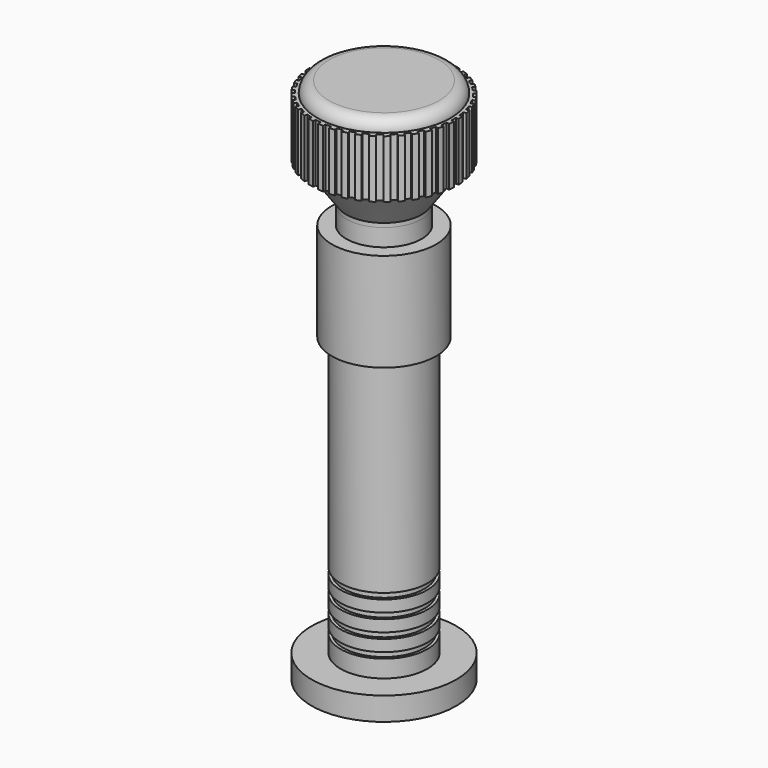
from build123d import *

# Parameters (mm, degrees)
F0_R             = 12.5
F1_DEPTH         = 4
F2_R             = 7.5
F3_DEPTH         = 3
F4_R             = 7
F5_DEPTH         = 1
F6_R             = 7.5
F7_DEPTH         = 2
F8_R             = 7
F9_DEPTH         = 1
F10_R            = 7.5
F11_DEPTH        = 2
F12_R            = 7
F13_DEPTH        = 1
F14_R            = 7.5
F15_DEPTH        = 2
F16_R            = 7
F17_DEPTH        = 1
F18_R            = 7.5
F19_DEPTH        = 35
F20_R            = 9
F21_DEPTH        = 17
F22_R            = 6.5
F23_DEPTH        = 3
F24_R            = 11
F25_DEPTH        = 7
F26_R            = 12.5
F27_DEPTH        = 10
F28_S6_R         = 6.5
F28_T7_DEPTH     = 17
F29_R            = 11.5
F30_DEPTH        = 2
F31_R            = 1.99999
F33_DEPTH        = 25
F33_COPIES_COUNT = 40
F34_R            = 2
F35_DEPTH        = 10


# Not quite as in the source:
# - a fillet or chamfer that OpenCascade refuses, or shapes differently, is made with other operations: its cross-section is extruded or revolved along the edge and cut away or added
# - a fillet or chamfer is up to 0.001 mm smaller than in the source, because OpenCascade refuses the exact size
# - a pattern or mirror of a feature is missing from the dataset's text; its kind, count and spacing are read off the source's solid


with BuildPart() as f1:
    # F0 (on Top) → F1 (new body)
    with BuildSketch(Plane.XY):
        Circle(F0_R)
    extrude(amount=F1_DEPTH)

    # F2 (on face) → F3 (join)
    with BuildSketch(Plane.XY.offset(4)):
        Circle(F2_R)
    extrude(amount=F3_DEPTH)

    # F4 (on face) → F5 (join)
    with BuildSketch(Plane.XY.offset(7)):
        Circle(F4_R)
    extrude(amount=F5_DEPTH)

    # F6 (on face) → F7 (join)
    with BuildSketch(Plane.XY.offset(8)):
        Circle(F6_R)
    extrude(amount=F7_DEPTH)

    # F8 (on face) → F9 (join)
    with BuildSketch(Plane.XY.offset(10)):
        Circle(F8_R)
    extrude(amount=F9_DEPTH)

    # F10 (on face) → F11 (join)
    with BuildSketch(Plane.XY.offset(11)):
        Circle(F10_R)
    extrude(amount=F11_DEPTH)

    # F12 (on face) → F13 (join)
    with BuildSketch(Plane.XY.offset(13)):
        Circle(F12_R)
    extrude(amount=F13_DEPTH)

    # F14 (on face) → F15 (join)
    with BuildSketch(Plane.XY.offset(14)):
        Circle(F14_R)
    extrude(amount=F15_DEPTH)

    # F16 (on face) → F17 (join)
    with BuildSketch(Plane.XY.offset(16)):
        Circle(F16_R)
    extrude(amount=F17_DEPTH)

    # F18 (on face) → F19 (join)
    with BuildSketch(Plane.XY.offset(17)):
        Circle(F18_R)
    extrude(amount=F19_DEPTH)

    # F20 (on face) → F21 (join)
    with BuildSketch(Plane.XY.offset(52)):
        Circle(F20_R)
    extrude(amount=F21_DEPTH)

    # F22 (on face) → F23 (join)
    with BuildSketch(Plane.XY.offset(69)):
        Circle(F22_R)
    extrude(amount=F23_DEPTH)

    # F24 (on face) → F25 (join)
    with BuildSketch(Plane.XY.offset(72)):
        Circle(F24_R)
    extrude(amount=F25_DEPTH)

    # F26 (on face) → F27 (join)
    with BuildSketch(Plane.XY.offset(79)):
        Circle(F26_R)
    extrude(amount=F27_DEPTH)

    # F28: chamfer of 7 x 5 on 1 edges, made by hand


with BuildPart() as f28_tool2:
    # F28_s3 → F28_t4 (revolve)
    with BuildSketch(Plane.XZ):
        Polygon((11, 79), (6, 72), (11, 72), align=None)
    revolve(axis=Axis((0, 0, 72), (0, 0, 1)))

    split(bisect_by=Plane.XY.offset(79), keep=Keep.BOTTOM)

    # F28_s6 → F28_t7 (cut, symmetric)
    with BuildSketch(Plane.XY.offset(75.5)):
        Circle(F28_S6_R)
    extrude(amount=F28_T7_DEPTH, both=True, mode=Mode.SUBTRACT)


with BuildPart() as f1_1:
    add(f1.part)

    # F28_t1: cut F28_tool2
    add(f28_tool2.part, mode=Mode.SUBTRACT)

    # F29 (on face) → F30 (join)
    with BuildSketch(Plane.XY.offset(89)):
        Circle(F29_R)
    extrude(amount=F30_DEPTH)

    # F31 (radius 2 in the source; OpenCascade refuses exactly that, so slightly less here)
    f31_edges = [f1_1.edges().sort_by_distance(p)[0] for p in [
        (-11.5, 0, 91),
    ]]
    fillet(f31_edges, radius=F31_R)

    # F32 (on face) → F33 (cut)
    with BuildSketch(Plane.XY.offset(89)):
        with BuildLine():
            ThreePointArc((0.5, 12.4899959968), (0, 12.5), (-0.5, 12.4899959968))
            Line((-0.5, 12.4899959968), (-0.5, 12))
            Line((-0.5, 12), (0.5, 12))
            Line((0.5, 12), (0.5, 12.4899959968))
        make_face()
    f33 = extrude(amount=-F33_DEPTH, mode=Mode.SUBTRACT)

    # F33_copies: F33 ×40 about axis
    f33_copies_axis = Axis((0, 0, 0), (0, 0, 1))
    for i in range(1, F33_COPIES_COUNT):
        add(f33.rotate(f33_copies_axis, i * 360 / F33_COPIES_COUNT), mode=Mode.SUBTRACT)

    # F34 (on face) → F35 (cut)
    with BuildSketch(Plane(origin=(0, 0, 0), x_dir=(1, 0, 0), z_dir=(0, 0, -1))):
        Circle(F34_R)
    extrude(amount=-F35_DEPTH, mode=Mode.SUBTRACT)


solid = f1_1.part
